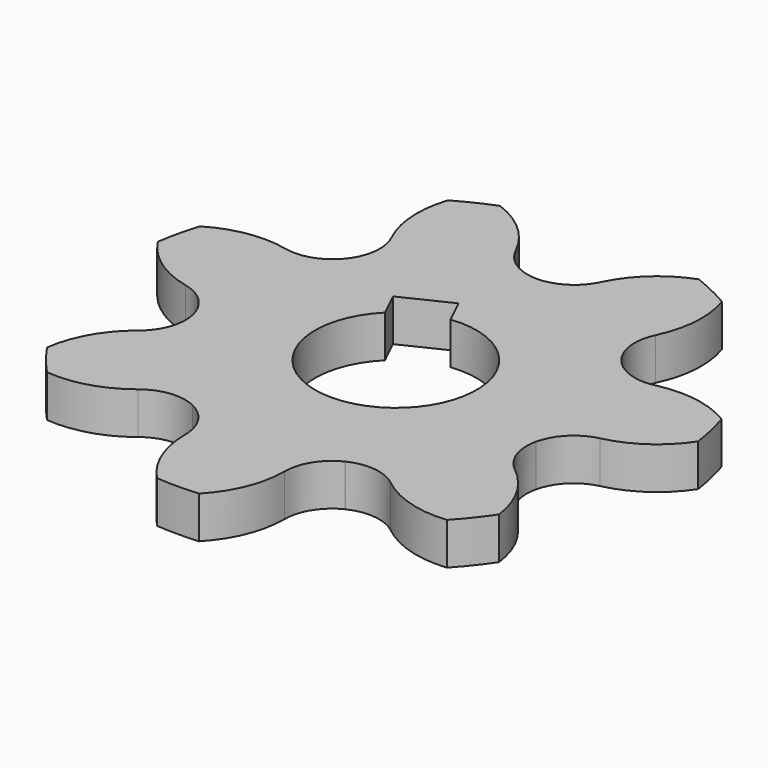
from build123d import *

# Parameters (mm, degrees)
F1_DEPTH = 8


# Not quite as in the source:
# - ends of sketch curves that miss each other by under 0.0002 mm in the source are joined


with BuildPart() as f1:
    # F0 (on Top) → F1 (new body)
    with BuildSketch(Plane.XY):
        with BuildLine():
            ThreePointArc((0.0173106263, 35.2915124556), (-6.457e-07, 35.2914532257), (-0.0173119996, 35.2914272939))
            ThreePointArc((-0.0173119996, 35.2914272939), (-4.7828415657, 36.6814206792), (-8.0865831016, 40.3864729511))
            ThreePointArc((-8.0865831016, 40.3864729511), (-12.5400209066, 46.3598395768), (-18.9133471994, 50.2192344565))
            ThreePointArc((-18.9133471994, 50.2192344565), (-22.5619545404, 48.6311460797), (-26.0784416984, 46.7687064797))
            ThreePointArc((-26.0784416984, 46.7687064797), (-27.0347490245, 39.379546207), (-25.1412558363, 32.173375079))
            ThreePointArc((-25.1412558363, 32.173375079), (-24.3043791298, 27.2803437578), (-26.1889642235, 22.6879091335))
            ThreePointArc((-26.1889642235, 22.6879091335), (-26.1997114341, 22.6743379832), (-26.2105512359, 22.6608403006))
            ThreePointArc((-26.2105512359, 22.6608403006), (-30.268483933, 19.8015929347), (-35.2250588486, 19.5286856632))
            ThreePointArc((-35.2250588486, 19.5286856632), (-42.6718988891, 19.7711813344), (-49.6630001039, 17.1946071711))
            ThreePointArc((-49.6630001039, 17.1946071711), (-50.6962513252, 13.3518540399), (-51.4326312922, 9.4413418946))
            ThreePointArc((-51.4326312922, 9.4413418946), (-46.2518013791, 4.086604184), (-39.4372158458, 1.0740226787))
            ThreePointArc((-39.4372158458, 1.0740226787), (-35.0899055663, -1.3224359394), (-32.6744151986, -5.6592003729))
            ThreePointArc((-32.6744151986, -5.6592003729), (-32.6705053342, -5.676064432), (-32.6666279149, -5.6929359805))
            ThreePointArc((-32.6666279149, -5.6929359805), (-32.9613409881, -10.648285961), (-35.8383477489, -14.6936473148))
            ThreePointArc((-35.8383477489, -14.6936473148), (-40.6709671644, -20.3646275254), (-43.0154005889, -27.4369580526))
            ThreePointArc((-43.0154005889, -27.4369580526), (-40.655237183, -30.6407045779), (-38.0570010523, -33.6545940487))
            ThreePointArc((-38.0570010523, -33.6545940487), (-30.6403035701, -32.942681267), (-24.0361481426, -29.4931378216))
            ThreePointArc((-24.0361481426, -29.4931378216), (-19.4520178261, -27.5884419734), (-14.5553656824, -28.4038640421))
            ThreePointArc((-14.5553656824, -28.4038640421), (-14.539742708, -28.4113209434), (-14.5241712519, -28.4188855039))
            ThreePointArc((-14.5241712519, -28.4188855039), (-10.8336363316, -31.7388351981), (-9.46463, -36.510411))
            ThreePointArc((-9.46463, -36.510411), (-8.0439677673, -43.8245030704), (-3.9763277521, -50.0669807595))
            ThreePointArc((-3.9763277521, -50.0669807595), (-4.985e-07, -50.219235), (3.9763270429, -50.066981559))
            ThreePointArc((3.9763270429, -50.066981559), (8.0439676368, -43.8245033926), (9.4646296494, -36.5104109994))
            ThreePointArc((9.4646296494, -36.5104109994), (10.8336355705, -31.738834816), (14.5241710621, -28.4188851093))
            ThreePointArc((14.5241710621, -28.4188851093), (14.5397421135, -28.4113207469), (14.555327686, -28.4037863488))
            ThreePointArc((14.555327686, -28.4037863488), (19.4520168261, -27.5884419734), (24.0361467636, -29.4931382964))
            ThreePointArc((24.0361467636, -29.4931382964), (30.6403030472, -32.9426814086), (38.0570009358, -33.6545933411))
            ThreePointArc((38.0570009358, -33.6545933411), (40.655237183, -30.6407045779), (43.0154002031, -27.436958138))
            ThreePointArc((43.0154002031, -27.436958138), (40.6709661644, -20.3646275254), (35.8383467951, -14.6936472574))
            ThreePointArc((35.8383467951, -14.6936472574), (32.9613408944, -10.6482856952), (32.6667108543, -5.6929547524))
            ThreePointArc((32.6667108543, -5.6929547524), (32.6705043598, -5.6760643215), (32.67441425, -5.659200152))
            ThreePointArc((32.67441425, -5.659200152), (35.0899046467, -1.3224358594), (39.4372149344, 1.0740222872))
            ThreePointArc((39.4372149344, 1.0740222872), (46.2518003791, 4.086604184), (51.4326310926, 9.4413419398))
            ThreePointArc((51.4326310926, 9.4413419398), (50.6962513088, 13.3518541117), (49.6629990471, 17.1946070146))
            ThreePointArc((49.6629990471, 17.1946070146), (42.6718983702, 19.7711812567), (35.2250588084, 19.5286858355))
            ThreePointArc((35.2250588084, 19.5286858355), (30.2684833934, 19.8015927747), (26.2105502359, 22.6608403006))
            ThreePointArc((26.2105502359, 22.6608403006), (26.1997106027, 22.6743373459), (26.1889636103, 22.687908644))
            ThreePointArc((26.1889636103, 22.687908644), (24.3043781641, 27.2803434477), (25.1412552893, 32.1733748607))
            ThreePointArc((25.1412552893, 32.1733748607), (27.0347490207, 39.3795461477), (26.0784413783, 46.768707126))
            ThreePointArc((26.0784413783, 46.768707126), (22.5619541507, 48.6311462674), (18.9133467528, 50.2192343669))
            ThreePointArc((18.9133467528, 50.2192343669), (12.5400199066, 46.3598395768), (8.0865821819, 40.3864729126))
            ThreePointArc((8.0865821819, 40.3864729126), (4.7828405657, 36.6814206792), (0.0173106263, 35.2915124556))
        make_face()
        with BuildLine():
            Line((-10.813517, 12.711431), (-13.133307, 17.528522))
            Line((-13.133307, 17.528522), (-4.123619, 21.867361))
            Line((-4.123619, 21.867361), (-1.803829, 17.050271))
            ThreePointArc((-1.803829, 17.050271), (6.6712619157, -12.0722441106), (-10.813517, 12.711431))
        make_face(mode=Mode.SUBTRACT)
    extrude(amount=-F1_DEPTH)


solid = f1.part
